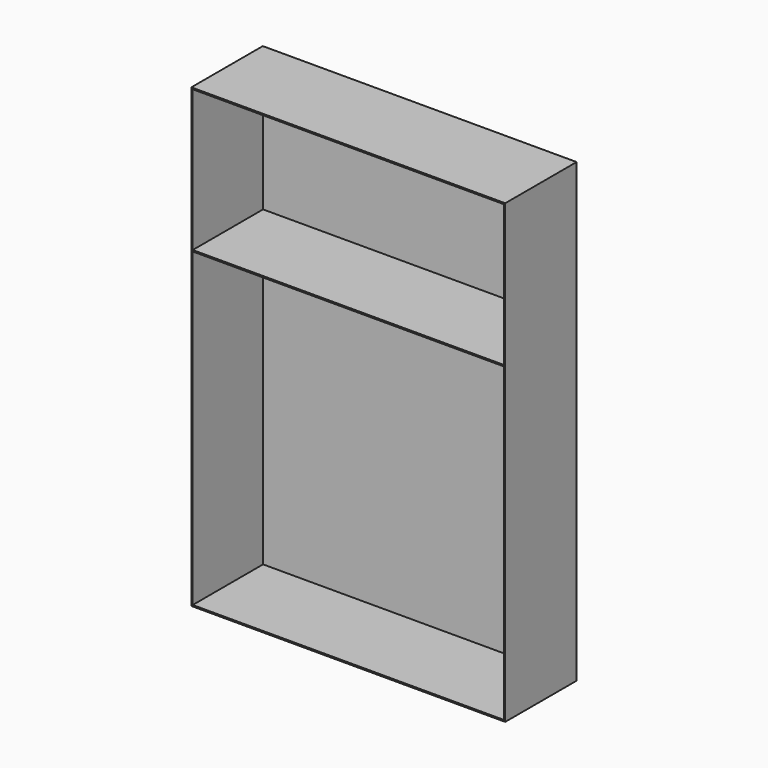
from build123d import *

# Parameters (mm, degrees)
F0_W     = 70.33
F0_H     = 70.33
F1_DEPTH = 20
F2_T     = -0.3
F0_H_2   = 32
F3_DEPTH = 20
F4_T     = -0.3


# Not quite as in the source:
# - a shell that OpenCascade refuses in one call is made with other operations: the cavity is built on its own and cut out


with BuildPart() as f1:
    # F0 (on Front) → F1 (new body)
    with BuildSketch(Plane.XZ):
        Rectangle(F0_W, F0_H)
    extrude(amount=F1_DEPTH)

    # F2
    f2_openings = [f1.faces().sort_by_distance(p)[0] for p in [
        (0, -20, 0),
    ]]
    offset(amount=F2_T, openings=f2_openings)

    # F0 (on Front) → F3 (join)
    with BuildSketch(Plane.XZ):
        with Locations((0, 51.165)):
            Rectangle(F0_W, F0_H_2)
    extrude(amount=F3_DEPTH)

    # F4: a shell. OpenCascade refuses it in one call, so the cavity is built on its own and cut out:
    # the body offset inwards by the wall thickness, plus a prism from it out through each open face.
    f4_core = offset(f1.part, amount=F4_T, kind=Kind.INTERSECTION, mode=Mode.PRIVATE)
    f4_exits = [f4_core.faces().sort_by_distance(p)[0] for p in [
        (0, -19.7, 51.015),
    ]]
    add(f4_core, mode=Mode.SUBTRACT)
    extrude(f4_exits, amount=-F4_T, mode=Mode.SUBTRACT)


solid = f1.part
